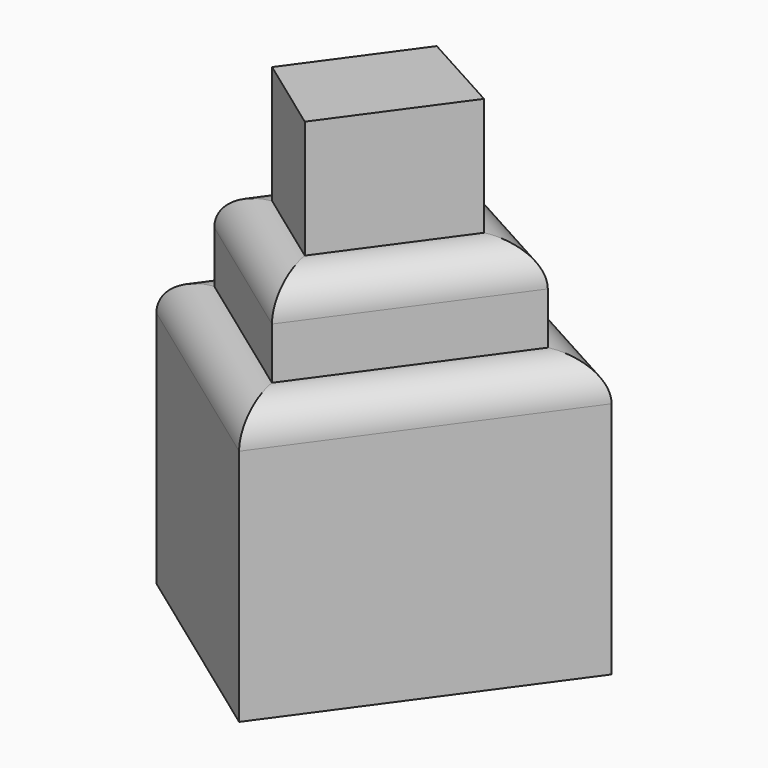
from build123d import *

# Parameters (mm, degrees)
F1_DEPTH = 38.0422770977
F2_R     = 5.08
F3_DEPTH = 12.232337147
F4_R     = 5.08
F5_DEPTH = 7.3413159698
F6_DEPTH = 8.9663118124


with BuildPart() as f1:
    # F0 (on Top) → F1 (new body)
    with BuildSketch(Plane.XY):
        Polygon((43.8701745906, -1.9375651716), (14.2481029034, 14.3980756402), (-7.7989399433, -16.04783535), (19.3933885201, -35.7388352654), align=None)
    extrude(amount=F1_DEPTH)

    # F2
    f2_edges = [f1.edges().sort_by_distance(p)[0] for p in [
        (31.631782, -18.8382, 38.042277),
        (29.059139, 6.230255, 38.042277),
        (3.224581, -0.82488, 38.042277),
        (5.797224, -25.893335, 38.042277),
    ]]
    fillet(f2_edges, radius=F2_R)

    # F3 (add): a face of the model
    f3_faces = [f1.faces().sort_by_distance(p)[0] for p in [
        (17.578761895, -9.9497918988, 38.0422770977),
    ]]
    extrude(f3_faces, amount=F3_DEPTH)

    # F4
    f4_edges = [f1.edges().sort_by_distance(p)[0] for p in [
        (7.511612, -3.566101, 50.274614),
        (8.776694, -21.77883, 50.274614),
        (27.322154, -16.128185, 50.274614),
        (26.057072, 2.084544, 50.274614),
    ]]
    fillet(f4_edges, radius=F4_R)

    # F5 (add): a face of the model
    f5_faces = [f1.faces().sort_by_distance(p)[0] for p in [
        (17.4849129571, -9.9130484235, 50.2746142447),
    ]]
    extrude(f5_faces, amount=F5_DEPTH)

    # F6 (add): a face of the model
    f6_faces = [f1.faces().sort_by_distance(p)[0] for p in [
        (17.4849129571, -9.9130484235, 57.6159302145),
    ]]
    extrude(f6_faces, amount=F6_DEPTH)


solid = f1.part
